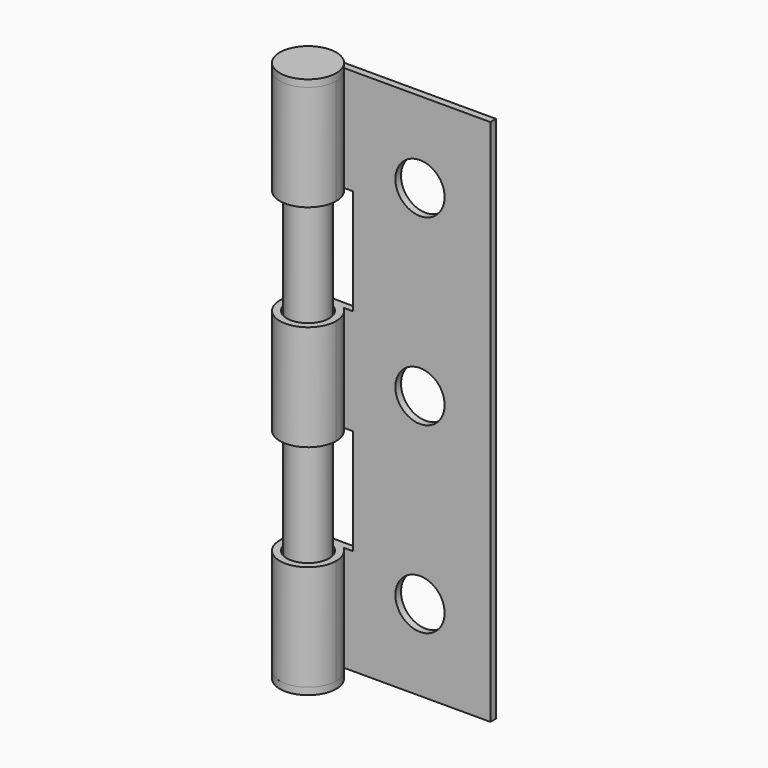
from build123d import *

# Parameters (mm, degrees)
F0_W          = 20
F0_H          = 75
F0_R          = 3.5
F1_DEPTH      = 1
F2_R          = 3
F3_DEPTH      = 75
F4_W          = 8
F4_H          = 15
F5_DEPTH      = 1.001
F5_DEPTH_BACK = 7.001
F6_R          = 2.75
F7_DEPTH      = 75
F8_R          = 4
F9_DEPTH      = 1
F10_R         = 4
F11_DEPTH     = 1


with BuildPart() as f1:
    # F0 (on Front) → F1 (new body)
    with BuildSketch(Plane.XZ):
        with Locations((-10, 0)):
            Rectangle(F0_W, F0_H)
        with Locations((-10, -26)):
            Circle(F0_R, mode=Mode.SUBTRACT)
        with Locations((-10, 0)):
            Circle(F0_R, mode=Mode.SUBTRACT)
        with Locations((-10, 26)):
            Circle(F0_R, mode=Mode.SUBTRACT)
    extrude(amount=F1_DEPTH)

    # F2 (on face) → F3 (join, through all)
    with BuildSketch(Plane(origin=(0, 0, -37.5), x_dir=(1, 0, 0), z_dir=(0, 0, -1))):
        with BuildLine():
            ThreePointArc((-20.8542486889, 1), (-19.8542486889, 2.3542486889), (-19.5, 4))
            ThreePointArc((-19.5, 4), (-26.3284271247, 6.8284271247), (-23.5, 0))
            ThreePointArc((-23.5, 0), (-22.0857864376, 0.2583426132), (-20.8542486889, 1))
        make_face()
        with Locations((-23.5, 4)):
            Circle(F2_R, mode=Mode.SUBTRACT)
        with BuildLine():
            ThreePointArc((-20.8542486889, 1), (-22.0857864376, 0.2583426132), (-23.5, 0))
            Line((-23.5, 0), (-20, 0))
            Line((-20, 0), (-20, 1))
            Line((-20, 1), (-20.8542486889, 1))
        make_face()
    extrude(amount=-F3_DEPTH)

    # F4 (on face) → F5 (cut, two sides)
    with BuildSketch(Plane.XZ.offset(1)) as f5_sk:
        with Locations((-23.5, -15)):
            Rectangle(F4_W, F4_H)
        with Locations((-23.5, 15)):
            Rectangle(F4_W, F4_H)
    extrude(amount=-F5_DEPTH, mode=Mode.SUBTRACT)
    extrude(f5_sk.sketch, amount=F5_DEPTH_BACK, mode=Mode.SUBTRACT)


with BuildPart() as f7:
    # F6 (on face) → F7 (new body, through all)
    with BuildSketch(Plane(origin=(0, 0, -37.5), x_dir=(1, 0, 0), z_dir=(0, 0, -1))):
        with Locations((-23.5, 4)):
            Circle(F6_R)
    extrude(amount=-F7_DEPTH)

    # F8 (on face) → F9 (join)
    with BuildSketch(Plane.XY.offset(37.5)):
        with Locations((-23.5, -4)):
            Circle(F8_R)
    extrude(amount=F9_DEPTH)

    # F10 (on face) → F11 (join)
    with BuildSketch(Plane(origin=(0, 0, -37.5), x_dir=(1, 0, 0), z_dir=(0, 0, -1))):
        with Locations((-23.5, 4)):
            Circle(F10_R)
    extrude(amount=F11_DEPTH)


solid = Compound([f1.part, f7.part])
